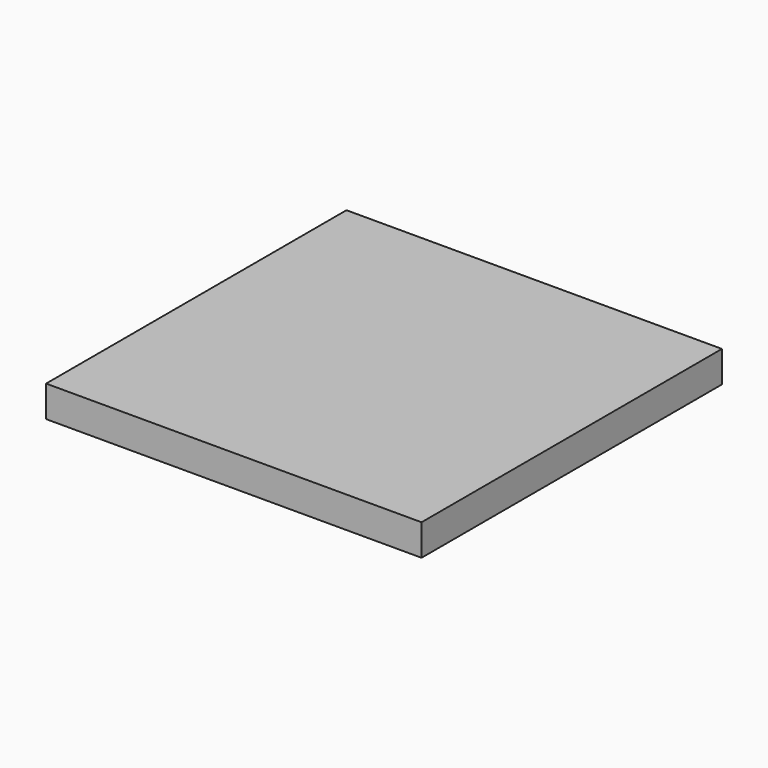
from build123d import *

# Parameters (mm, degrees)
F0_W     = 1219.2
F0_H     = 1219.2
F1_DEPTH = 101.6


# Not quite as in the source:
# - the program builds the solid bodies; features that only make, move or delete a surface that nothing else refers to are left out


with BuildPart() as f1:
    # F0 (on Top) → F1 (new body)
    with BuildSketch(Plane.XY):
        with Locations((-609.6, 609.6)):
            Rectangle(F0_W, F0_H)
    extrude(amount=F1_DEPTH)


solid = f1.part
